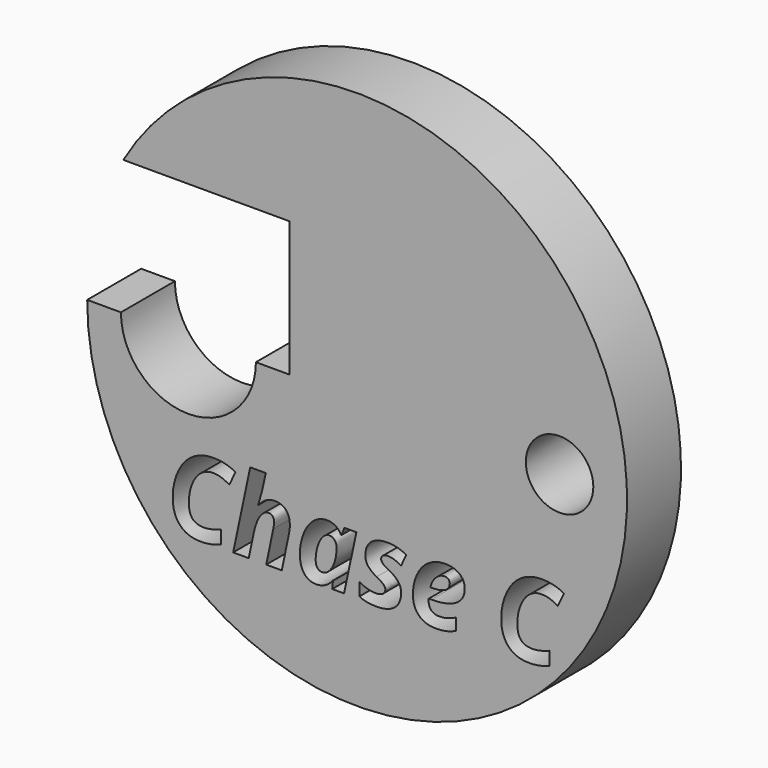
from build123d import *

# Parameters (mm, degrees)
F1_DEPTH     = 3.175
F2_R         = 1.5875
F3_DEPTH     = 3.176
F4_TEXT_SIZE = 4.9849034339
F5_DEPTH     = 3.176


# Not quite as in the source:
# - Text() gives the source's letters only with a copy of the font that has no kerning and outlines rounded to 1/6400 em; it was checked with that copy


with BuildPart() as f1:
    # F0 (on Front) → F1 (new body)
    with BuildSketch(Plane.XZ):
        with BuildLine():
            Line((-11.1125, 0), (-12.7, 0))
            ThreePointArc((-12.7, 0), (12.2672579939, -3.2870018728), (-10.9985226281, 6.35))
            Line((-10.9985226281, 6.35), (-3.175, 6.35))
            Line((-3.175, 6.35), (-3.175, 0))
            Line((-3.175, 0), (-4.7625, 0))
            ThreePointArc((-4.7625, 0), (-7.9375, -3.175), (-11.1125, 0))
        make_face()
    extrude(amount=F1_DEPTH)

    # F2 (on Front) → F3 (cut, through all)
    with BuildSketch(Plane.XZ):
        with Locations((9.525, 0)):
            Circle(F2_R)
    extrude(amount=F3_DEPTH, mode=Mode.SUBTRACT)

    # F4 (on Front) → F5 (cut, through all)
    with BuildSketch(Plane.XZ):
        with Locations((-8.9728264138, -8.2273911685)):
            Text('Chase C', F4_TEXT_SIZE, font='Open Sans', font_style=FontStyle.BOLDITALIC, text_align=(TextAlign.LEFT, TextAlign.BOTTOM))
    extrude(amount=F5_DEPTH, mode=Mode.SUBTRACT)


solid = f1.part
